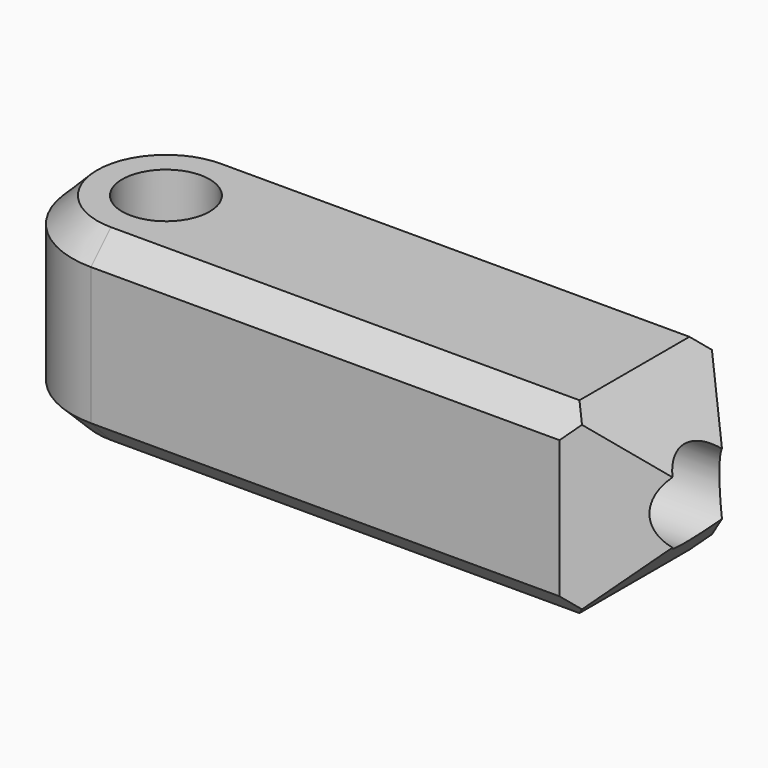
from build123d import *

# Parameters (mm, degrees)
F0_W        = 50
F0_H        = 15
F1_DEPTH    = 15
F2_R        = 7.49999
F3_R        = 3.5
F4_DEPTH    = 25
F6_DEPTH    = 30
F7_SIZE     = 2
F8_T1_DEPTH = 36.7168298797
F8_T3_DEPTH = 36.7168298797


# Not quite as in the source:
# - a fillet or chamfer that OpenCascade refuses, or shapes differently, is made with other operations: its cross-section is extruded or revolved along the edge and cut away or added
# - a fillet or chamfer is up to 0.001 mm smaller than in the source, because OpenCascade refuses the exact size


with BuildPart() as f1:
    # F0 (on Top) → F1 (new body)
    with BuildSketch(Plane.XY):
        with Locations((-34.3210311607, 15.3476024792)):
            Rectangle(F0_W, F0_H)
    extrude(amount=F1_DEPTH)

    # F2 (radius 7.5 in the source; OpenCascade refuses exactly that, so slightly less here)
    f2_edges = [f1.edges().sort_by_distance(p)[0] for p in [
        (-59.321031, 22.847602, 7.5),
        (-59.321031, 7.847602, 7.5),
    ]]
    fillet(f2_edges, radius=F2_R)

    # F3 (on face) → F4 (cut)
    with BuildSketch(Plane.XY.offset(15)):
        with Locations((-51.8210311607, 15.3476024792)):
            Circle(F3_R)
    extrude(amount=-F4_DEPTH, mode=Mode.SUBTRACT)

    # F5 (on face) → F6 (cut)
    with BuildSketch(Plane.YZ.offset(-9.3210311607)):
        with BuildLine():
            ThreePointArc((18.8476024792, 7.5), (15.3476024792, 11), (11.8476024792, 7.5))
            ThreePointArc((11.8476024792, 7.5), (15.3476024792, 4), (18.8476024792, 7.5))
        make_face()
    extrude(amount=-F6_DEPTH, mode=Mode.SUBTRACT)

    # F7
    f7_edges = [f1.edges().sort_by_distance(p)[0] for p in [
        (-30.571036, 7.847602, 15),
        (-30.571036, 7.847602, 0),
    ]]
    chamfer(f7_edges, length=F7_SIZE)

    # F8: chamfer of 5 on 4 edges, made by hand

    # F8_s2 → F8_t1 (cut)
    with BuildSketch(Plane.XZ.offset(-33.706017419)):
        Polygon((-9.3210311607, 10), (-14.3210311607, 15), (-9.3210311607, 15), align=None)
        Polygon((-9.3210311607, 5), (-14.3210311607, 0), (-9.3210311607, 0), align=None)
    extrude(amount=F8_T1_DEPTH, mode=Mode.SUBTRACT)

    # F8_s4 → F8_t3 (cut)
    with BuildSketch(Plane.XY.offset(-10.8584149398)):
        Polygon((-9.3210311607, 12.8476024792), (-14.3210311607, 7.8476024792), (-9.3210311607, 7.8476024792), align=None)
        Polygon((-14.3210311607, 22.8476024792), (-9.3210311607, 17.8476024792), (-9.3210311607, 22.8476024792), align=None)
    extrude(amount=F8_T3_DEPTH, mode=Mode.SUBTRACT)


solid = f1.part
